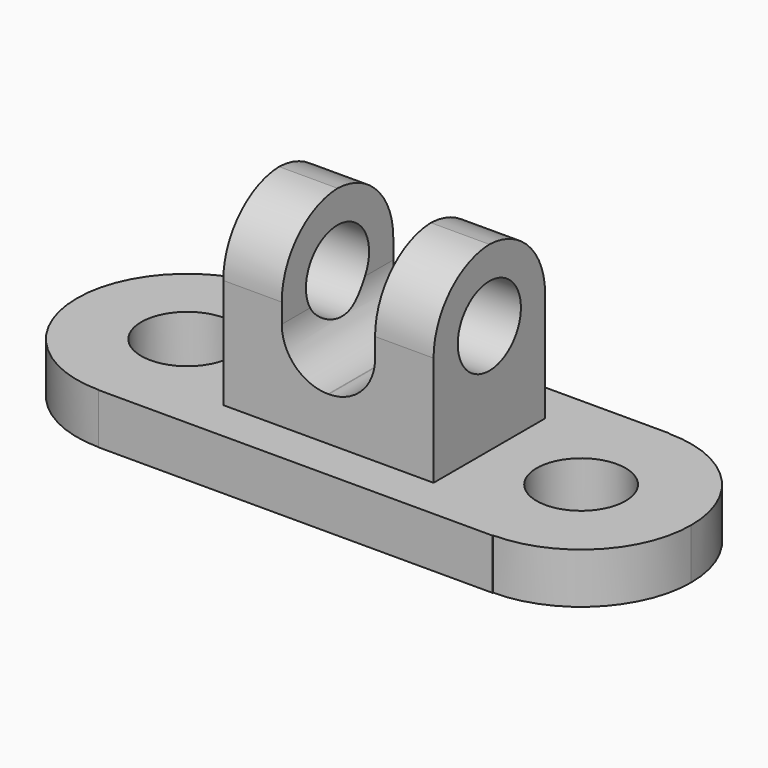
from build123d import *

# Parameters (mm, degrees)
F1_DEPTH    = 25.4
F2_W        = 105.8882400393
F2_H        = 70.1928213239
F3_DEPTH    = 55.88
F4_W        = 46.9851754606
F4_H        = 70.1928213239
F5_DEPTH    = 33.782
F6_R        = 23.301989304
F7_DEPTH    = 35.56
F8_T1_DEPTH = 210.348554518
F8_T3_DEPTH = 210.348554518
F9_R        = 19.8729907894
F10_DEPTH   = 207.5309093164


# Not quite as in the source:
# - a fillet or chamfer that OpenCascade refuses, or shapes differently, is made with other operations: its cross-section is extruded or revolved along the edge and cut away or added


with BuildPart() as f1:
    # F0 (on Top) → F1 (new body)
    with BuildSketch(Plane.XY):
        with BuildLine():
            Line((-99.153496325, -55.7124875486), (99.153496325, -55.7124875486))
            Line((99.153496325, -55.7124875486), (99.153496325, -55.4322929717))
            ThreePointArc((99.153496325, -55.4322929717), (43.7212033534, 0), (99.153496325, 55.4322929717))
            Line((99.153496325, 55.4322929717), (99.153496325, 55.7124875486))
            Line((99.153496325, 55.7124875486), (-99.153496325, 55.7124875486))
            Line((-99.153496325, 55.7124875486), (-99.153496325, 55.5695868493))
            ThreePointArc((-99.153496325, 55.5695868493), (-59.8598646362, 39.2936316888), (-43.5839094758, 0))
            ThreePointArc((-43.5839094758, 0), (-59.8598646362, -39.2936316888), (-99.153496325, -55.5695868493))
            Line((-99.153496325, -55.5695868493), (-99.153496325, -55.7124875486))
        make_face()
        with BuildLine():
            Line((99.153496325, -22.3866111857), (99.153496325, -55.4322929717))
            ThreePointArc((99.153496325, -55.4322929717), (138.350046582, -39.196550257), (154.5857892967, 0))
            ThreePointArc((154.5857892967, 0), (138.350046582, 39.196550257), (99.153496325, 55.4322929717))
            Line((99.153496325, 55.4322929717), (99.153496325, 22.3866111857))
            ThreePointArc((99.153496325, 22.3866111857), (114.9832209022, 15.8297245772), (121.5401075107, 0))
            ThreePointArc((121.5401075107, 0), (114.9832209022, -15.8297245772), (99.153496325, -22.3866111857))
        make_face()
        with BuildLine():
            ThreePointArc((-99.153496325, 55.5695868493), (-154.7230831743, 0), (-99.153496325, -55.5695868493))
            Line((-99.153496325, -55.5695868493), (-99.153496325, -23.1719717835))
            ThreePointArc((-99.153496325, -23.1719717835), (-122.3254681085, 0), (-99.153496325, 23.1719717835))
            Line((-99.153496325, 23.1719717835), (-99.153496325, 55.5695868493))
        make_face()
        with BuildLine():
            ThreePointArc((99.153496325, 55.4322929717), (43.7212033534, 0), (99.153496325, -55.4322929717))
            Line((99.153496325, -55.4322929717), (99.153496325, -22.3866111857))
            ThreePointArc((99.153496325, -22.3866111857), (76.7668851393, 0), (99.153496325, 22.3866111857))
            Line((99.153496325, 22.3866111857), (99.153496325, 55.4322929717))
        make_face()
        with BuildLine():
            Line((-99.153496325, -23.1719717835), (-99.153496325, -55.5695868493))
            ThreePointArc((-99.153496325, -55.5695868493), (-59.8598646362, -39.2936316888), (-43.5839094758, 0))
            ThreePointArc((-43.5839094758, 0), (-59.8598646362, 39.2936316888), (-99.153496325, 55.5695868493))
            Line((-99.153496325, 55.5695868493), (-99.153496325, 23.1719717835))
            ThreePointArc((-99.153496325, 23.1719717835), (-82.7684379434, 16.3850583816), (-75.9815245415, 0))
            ThreePointArc((-75.9815245415, 0), (-82.7684379434, -16.3850583816), (-99.153496325, -23.1719717835))
        make_face()
    extrude(amount=F1_DEPTH)

    # F2 (on face) → F3 (join)
    with BuildSketch(Plane.XY.offset(25.4)):
        Rectangle(F2_W, F2_H)
    extrude(amount=F3_DEPTH)

    # F4 (on face) → F5 (cut)
    with BuildSketch(Plane.XY.offset(81.28)):
        Rectangle(F4_W, F4_H)
    extrude(amount=-F5_DEPTH, mode=Mode.SUBTRACT)

    # F6
    f6_edges = [f1.edges().sort_by_distance(p)[0] for p in [
        (-23.492588, 0, 47.498),
        (23.492588, 0, 47.498),
    ]]
    fillet(f6_edges, radius=F6_R)

    # F7 (add): faces of the model
    f7_faces = [f1.faces().sort_by_distance(p)[0] for p in [
        (-38.218353875, 0, 81.28),
        (38.218353875, 0, 81.28),
    ]]
    extrude(f7_faces, amount=F7_DEPTH)

    # F8: fillet of radius 36.1794044457 on 4 edges, made by hand

    # F8_s2 → F8_t1 (cut)
    with BuildSketch(Plane.YZ.offset(-143.392631134)):
        with BuildLine():
            ThreePointArc((-35.0964106619, 80.6605955543), (-24.4997084391, 106.2432977771), (1.0829937838, 116.84))
            Line((1.0829937838, 116.84), (-35.0964106619, 116.84))
            Line((-35.0964106619, 116.84), (-35.0964106619, 80.6605955543))
        make_face()
        with BuildLine():
            ThreePointArc((35.0964106619, 80.6605955543), (24.4997084391, 106.2432977771), (-1.0829937838, 116.84))
            Line((-1.0829937838, 116.84), (35.0964106619, 116.84))
            Line((35.0964106619, 116.84), (35.0964106619, 80.6605955543))
        make_face()
    extrude(amount=F8_T1_DEPTH, mode=Mode.SUBTRACT)

    # F8_s4 → F8_t3 (cut)
    with BuildSketch(Plane.YZ.offset(-66.955923384)):
        with BuildLine():
            ThreePointArc((-35.0964106619, 80.6605955543), (-24.4997084391, 106.2432977771), (1.0829937838, 116.84))
            Line((1.0829937838, 116.84), (-35.0964106619, 116.84))
            Line((-35.0964106619, 116.84), (-35.0964106619, 80.6605955543))
        make_face()
        with BuildLine():
            ThreePointArc((35.0964106619, 80.6605955543), (24.4997084391, 106.2432977771), (-1.0829937838, 116.84))
            Line((-1.0829937838, 116.84), (35.0964106619, 116.84))
            Line((35.0964106619, 116.84), (35.0964106619, 80.6605955543))
        make_face()
    extrude(amount=F8_T3_DEPTH, mode=Mode.SUBTRACT)

    # F9 (on face) → F10 (cut, through all)
    with BuildSketch(Plane(origin=(-52.9441200197, 0, 0), x_dir=(0, -1, 0), z_dir=(-1, 0, 0))):
        with Locations((0, 80.6605955543)):
            Circle(F9_R)
    extrude(amount=-F10_DEPTH, mode=Mode.SUBTRACT)


solid = f1.part
